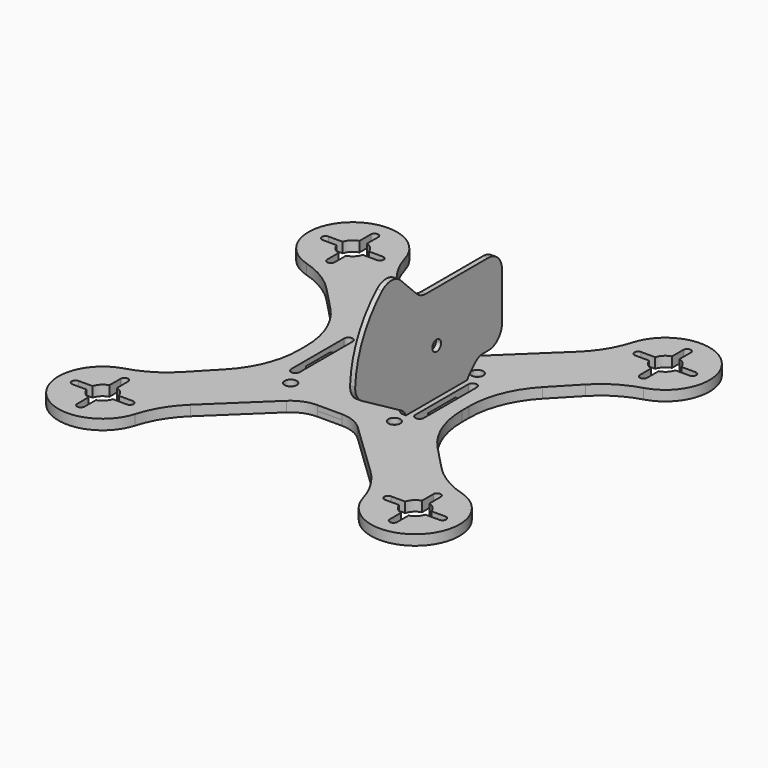
from build123d import *

# Parameters (mm, degrees)
F0_R     = 1.75
F0_W     = 2.5
F0_H     = 22
F0_R_2   = 5
F1_DEPTH = 3
F2_R     = 1.75
F2_R_2   = 8
F2_R_3   = 3.5
F3_DEPTH = 1.5
F4_R     = 1.24999
F6_W     = 11.5
F6_H     = 1.5
F6_R     = 1.6
F7_DEPTH = 1.5


# Not quite as in the source:
# - a fillet or chamfer is up to 0.001 mm smaller than in the source, because OpenCascade refuses the exact size


with BuildPart() as f1:
    # F0 (on Top) → F1 (new body)
    with BuildSketch(Plane.XY):
        with BuildLine():
            ThreePointArc((38.0929628562, 26.4985966632), (43.3866280041, 30.7474383597), (49.5996537841, 33.4812739649))
            ThreePointArc((49.5996537841, 33.4812739649), (55.1543289326, 55.1543289326), (33.4812739649, 49.5996537841))
            ThreePointArc((33.4812739649, 49.5996537841), (30.7474383597, 43.3866280041), (26.4985966632, 38.0929628562))
            Line((26.4985966632, 38.0929628562), (10.4972371837, 22.7761088685))
            ThreePointArc((10.4972371837, 22.7761088685), (7.3080296231, 20.7199431221), (3.5823693672, 20))
            Line((3.5823693672, 20), (-3.5823693672, 20))
            ThreePointArc((-3.5823693672, 20), (-7.3080296231, 20.7199431221), (-10.4972371837, 22.7761088685))
            Line((-10.4972371837, 22.7761088685), (-26.4985966632, 38.0929628562))
            ThreePointArc((-26.4985966632, 38.0929628562), (-30.7474383597, 43.3866280041), (-33.4812739649, 49.5996537841))
            ThreePointArc((-33.4812739649, 49.5996537841), (-55.1543289326, 55.1543289326), (-49.5996537841, 33.4812739649))
            ThreePointArc((-49.5996537841, 33.4812739649), (-43.3866280041, 30.7474383597), (-38.0929628562, 26.4985966632))
            Line((-38.0929628562, 26.4985966632), (-31.217883058, 19.3162716643))
            ThreePointArc((-31.217883058, 19.3162716643), (-25.8718521174, 11.0243320067), (-24, 1.3376153414))
            Line((-24, 1.3376153414), (-24, -1.3376153414))
            ThreePointArc((-24, -1.3376153414), (-25.8718521174, -11.0243320067), (-31.217883058, -19.3162716643))
            Line((-31.217883058, -19.3162716643), (-38.0929628562, -26.4985966632))
            ThreePointArc((-38.0929628562, -26.4985966632), (-43.3866280041, -30.7474383597), (-49.5996537841, -33.4812739649))
            ThreePointArc((-49.5996537841, -33.4812739649), (-55.1543289326, -55.1543289326), (-33.4812739649, -49.5996537841))
            ThreePointArc((-33.4812739649, -49.5996537841), (-30.7474383597, -43.3866280041), (-26.4985966632, -38.0929628562))
            Line((-26.4985966632, -38.0929628562), (-10.4972371837, -22.7761088685))
            ThreePointArc((-10.4972371837, -22.7761088685), (-7.3080296231, -20.7199431221), (-3.5823693672, -20))
            Line((-3.5823693672, -20), (3.5823693672, -20))
            ThreePointArc((3.5823693672, -20), (7.3080296231, -20.7199431221), (10.4972371837, -22.7761088685))
            Line((10.4972371837, -22.7761088685), (26.4985966632, -38.0929628562))
            ThreePointArc((26.4985966632, -38.0929628562), (30.7474383597, -43.3866280041), (33.4812739649, -49.5996537841))
            ThreePointArc((33.4812739649, -49.5996537841), (55.1543289326, -55.1543289326), (49.5996537841, -33.4812739649))
            ThreePointArc((49.5996537841, -33.4812739649), (43.3866280041, -30.7474383597), (38.0929628562, -26.4985966632))
            Line((38.0929628562, -26.4985966632), (31.217883058, -19.3162716643))
            ThreePointArc((31.217883058, -19.3162716643), (25.8718521174, -11.0243320067), (24, -1.3376153414))
            Line((24, -1.3376153414), (24, 1.3376153414))
            ThreePointArc((24, 1.3376153414), (25.8718521174, 11.0243320067), (31.217883058, 19.3162716643))
            Line((31.217883058, 19.3162716643), (38.0929628562, 26.4985966632))
        make_face()
        with BuildLine():
            Line((-42.1161638725, -44.8619407771), (-37.9619407771, -44.8619407771))
            ThreePointArc((-37.9619407771, -44.8619407771), (-36.8619407771, -45.9619407771), (-37.9619407771, -47.0619407771))
            Line((-37.9619407771, -47.0619407771), (-42.1161638725, -47.0619407771))
            ThreePointArc((-42.1161638725, -47.0619407771), (-43.1335136524, -48.7903679019), (-44.8619407771, -49.8077176817))
            Line((-44.8619407771, -49.8077176817), (-44.8619407771, -53.9619407771))
            ThreePointArc((-44.8619407771, -53.9619407771), (-45.9619407771, -55.0619407771), (-47.0619407771, -53.9619407771))
            Line((-47.0619407771, -53.9619407771), (-47.0619407771, -49.8077176817))
            ThreePointArc((-47.0619407771, -49.8077176817), (-48.7903679019, -48.7903679019), (-49.8077176817, -47.0619407771))
            Line((-49.8077176817, -47.0619407771), (-53.9619407771, -47.0619407771))
            ThreePointArc((-53.9619407771, -47.0619407771), (-55.0619407771, -45.9619407771), (-53.9619407771, -44.8619407771))
            Line((-53.9619407771, -44.8619407771), (-49.8077176817, -44.8619407771))
            ThreePointArc((-49.8077176817, -44.8619407771), (-48.7903679019, -43.1335136524), (-47.0619407771, -42.1161638725))
            Line((-47.0619407771, -42.1161638725), (-47.0619407771, -37.9619407771))
            ThreePointArc((-47.0619407771, -37.9619407771), (-45.9619407771, -36.8619407771), (-44.8619407771, -37.9619407771))
            Line((-44.8619407771, -37.9619407771), (-44.8619407771, -42.1161638725))
            ThreePointArc((-44.8619407771, -42.1161638725), (-43.1335136524, -43.1335136524), (-42.1161638725, -44.8619407771))
        make_face(mode=Mode.SUBTRACT)
        with Locations((-15.25, -15.25)):
            Circle(F0_R, mode=Mode.SUBTRACT)
        with BuildLine():
            Line((44.8619407771, -42.1161638725), (44.8619407771, -37.9619407771))
            ThreePointArc((44.8619407771, -37.9619407771), (45.9619407771, -36.8619407771), (47.0619407771, -37.9619407771))
            Line((47.0619407771, -37.9619407771), (47.0619407771, -42.1161638725))
            ThreePointArc((47.0619407771, -42.1161638725), (48.7903679019, -43.1335136524), (49.8077176817, -44.8619407771))
            Line((49.8077176817, -44.8619407771), (53.9619407771, -44.8619407771))
            ThreePointArc((53.9619407771, -44.8619407771), (55.0619407771, -45.9619407771), (53.9619407771, -47.0619407771))
            Line((53.9619407771, -47.0619407771), (49.8077176817, -47.0619407771))
            ThreePointArc((49.8077176817, -47.0619407771), (48.7903679019, -48.7903679019), (47.0619407771, -49.8077176817))
            Line((47.0619407771, -49.8077176817), (47.0619407771, -53.9619407771))
            ThreePointArc((47.0619407771, -53.9619407771), (45.9619407771, -55.0619407771), (44.8619407771, -53.9619407771))
            Line((44.8619407771, -53.9619407771), (44.8619407771, -49.8077176817))
            ThreePointArc((44.8619407771, -49.8077176817), (43.1335136524, -48.7903679019), (42.1161638725, -47.0619407771))
            Line((42.1161638725, -47.0619407771), (37.9619407771, -47.0619407771))
            ThreePointArc((37.9619407771, -47.0619407771), (36.8619407771, -45.9619407771), (37.9619407771, -44.8619407771))
            Line((37.9619407771, -44.8619407771), (42.1161638725, -44.8619407771))
            ThreePointArc((42.1161638725, -44.8619407771), (43.1335136524, -43.1335136524), (44.8619407771, -42.1161638725))
        make_face(mode=Mode.SUBTRACT)
        with Locations((15.25, -15.25)):
            Circle(F0_R, mode=Mode.SUBTRACT)
        with Locations((-18.25, 0)):
            Rectangle(F0_W, F0_H, mode=Mode.SUBTRACT)
        with Locations((-15.25, 15.25)):
            Circle(F0_R, mode=Mode.SUBTRACT)
        with BuildLine():
            Line((-44.8619407771, 42.1161638725), (-44.8619407771, 37.9619407771))
            ThreePointArc((-44.8619407771, 37.9619407771), (-45.9619407771, 36.8619407771), (-47.0619407771, 37.9619407771))
            Line((-47.0619407771, 37.9619407771), (-47.0619407771, 42.1161638725))
            ThreePointArc((-47.0619407771, 42.1161638725), (-48.7903679019, 43.1335136524), (-49.8077176817, 44.8619407771))
            Line((-49.8077176817, 44.8619407771), (-53.9619407771, 44.8619407771))
            ThreePointArc((-53.9619407771, 44.8619407771), (-55.0619407771, 45.9619407771), (-53.9619407771, 47.0619407771))
            Line((-53.9619407771, 47.0619407771), (-49.8077176817, 47.0619407771))
            ThreePointArc((-49.8077176817, 47.0619407771), (-48.7903679019, 48.7903679019), (-47.0619407771, 49.8077176817))
            Line((-47.0619407771, 49.8077176817), (-47.0619407771, 53.9619407771))
            ThreePointArc((-47.0619407771, 53.9619407771), (-45.9619407771, 55.0619407771), (-44.8619407771, 53.9619407771))
            Line((-44.8619407771, 53.9619407771), (-44.8619407771, 49.8077176817))
            ThreePointArc((-44.8619407771, 49.8077176817), (-43.1335136524, 48.7903679019), (-42.1161638725, 47.0619407771))
            Line((-42.1161638725, 47.0619407771), (-37.9619407771, 47.0619407771))
            ThreePointArc((-37.9619407771, 47.0619407771), (-36.8619407771, 45.9619407771), (-37.9619407771, 44.8619407771))
            Line((-37.9619407771, 44.8619407771), (-42.1161638725, 44.8619407771))
            ThreePointArc((-42.1161638725, 44.8619407771), (-43.1335136524, 43.1335136524), (-44.8619407771, 42.1161638725))
        make_face(mode=Mode.SUBTRACT)
        Circle(F0_R_2, mode=Mode.SUBTRACT)
        with Locations((18.25, 0)):
            Rectangle(F0_W, F0_H, mode=Mode.SUBTRACT)
        with Locations((15.25, 15.25)):
            Circle(F0_R, mode=Mode.SUBTRACT)
        with BuildLine():
            ThreePointArc((42.1161638725, 47.0619407771), (43.1335136524, 48.7903679019), (44.8619407771, 49.8077176817))
            Line((44.8619407771, 49.8077176817), (44.8619407771, 53.9619407771))
            ThreePointArc((44.8619407771, 53.9619407771), (45.9619407771, 55.0619407771), (47.0619407771, 53.9619407771))
            Line((47.0619407771, 53.9619407771), (47.0619407771, 49.8077176817))
            ThreePointArc((47.0619407771, 49.8077176817), (48.7903679019, 48.7903679019), (49.8077176817, 47.0619407771))
            Line((49.8077176817, 47.0619407771), (53.9619407771, 47.0619407771))
            ThreePointArc((53.9619407771, 47.0619407771), (55.0619407771, 45.9619407771), (53.9619407771, 44.8619407771))
            Line((53.9619407771, 44.8619407771), (49.8077176817, 44.8619407771))
            ThreePointArc((49.8077176817, 44.8619407771), (48.7903679019, 43.1335136524), (47.0619407771, 42.1161638725))
            Line((47.0619407771, 42.1161638725), (47.0619407771, 37.9619407771))
            ThreePointArc((47.0619407771, 37.9619407771), (45.9619407771, 36.8619407771), (44.8619407771, 37.9619407771))
            Line((44.8619407771, 37.9619407771), (44.8619407771, 42.1161638725))
            ThreePointArc((44.8619407771, 42.1161638725), (43.1335136524, 43.1335136524), (42.1161638725, 44.8619407771))
            Line((42.1161638725, 44.8619407771), (37.9619407771, 44.8619407771))
            ThreePointArc((37.9619407771, 44.8619407771), (36.8619407771, 45.9619407771), (37.9619407771, 47.0619407771))
            Line((37.9619407771, 47.0619407771), (42.1161638725, 47.0619407771))
        make_face(mode=Mode.SUBTRACT)
    extrude(amount=F1_DEPTH)

    # F4 (radius 1.25 in the source; OpenCascade refuses exactly that, so slightly less here)
    f4_edges = [f1.edges().sort_by_distance(p)[0] for p in [
        (-19.5, 11, 1.5),
        (-17, 11, 1.5),
        (-19.5, -11, 1.5),
        (-17, -11, 1.5),
        (17, -11, 1.5),
        (19.5, -11, 1.5),
        (17, 11, 1.5),
        (19.5, 11, 1.5),
    ]]
    fillet(f4_edges, radius=F4_R)


with BuildPart() as f3:
    # F2 (on Top) → F3 (new body)
    with BuildSketch(Plane.XY):
        with BuildLine():
            Line((-10.9087121146, 20), (-15, 20))
            ThreePointArc((-15, 20), (-18.5355339059, 18.5355339059), (-20, 15))
            Line((-20, 15), (-20, 13))
            ThreePointArc((-20, 13), (-19.4142135624, 11.5857864376), (-18, 11))
            Line((-18, 11), (-14, 11))
            ThreePointArc((-14, 11), (-13.5, 10.5), (-14, 10))
            Line((-14, 10), (-14, 6))
            ThreePointArc((-14, 6), (-13.5, 5.5), (-14, 5))
            Line((-14, 5), (-18, 5))
            ThreePointArc((-18, 5), (-19.4142135624, 4.4142135624), (-20, 3))
            Line((-20, 3), (-20, -3))
            ThreePointArc((-20, -3), (-19.4142135624, -4.4142135624), (-18, -5))
            Line((-18, -5), (-14, -5))
            ThreePointArc((-14, -5), (-13.5, -5.5), (-14, -6))
            Line((-14, -6), (-14, -10))
            ThreePointArc((-14, -10), (-13.5, -10.5), (-14, -11))
            Line((-14, -11), (-18, -11))
            ThreePointArc((-18, -11), (-19.4142135624, -11.5857864376), (-20, -13))
            Line((-20, -13), (-20, -15))
            ThreePointArc((-20, -15), (-18.5355339059, -18.5355339059), (-15, -20))
            Line((-15, -20), (15, -20))
            ThreePointArc((15, -20), (18.5355339059, -18.5355339059), (20, -15))
            Line((20, -15), (20, -13))
            ThreePointArc((20, -13), (19.4142135624, -11.5857864376), (18, -11))
            Line((18, -11), (14, -11))
            ThreePointArc((14, -11), (13.5, -10.5), (14, -10))
            Line((14, -10), (14, -6))
            ThreePointArc((14, -6), (13.5, -5.5), (14, -5))
            Line((14, -5), (18, -5))
            ThreePointArc((18, -5), (19.4142135624, -4.4142135624), (20, -3))
            Line((20, -3), (20, 3))
            ThreePointArc((20, 3), (19.4142135624, 4.4142135624), (18, 5))
            Line((18, 5), (14, 5))
            ThreePointArc((14, 5), (13.5, 5.5), (14, 6))
            Line((14, 6), (14, 10))
            ThreePointArc((14, 10), (13.5, 10.5), (14, 11))
            Line((14, 11), (18, 11))
            ThreePointArc((18, 11), (19.4142135624, 11.5857864376), (20, 13))
            Line((20, 13), (20, 15))
            ThreePointArc((20, 15), (18.5355339059, 18.5355339059), (15, 20))
            Line((15, 20), (10.9087121146, 20))
            ThreePointArc((10.9087121146, 20), (8.2084034903, 20.7918729423), (6.3634154002, 22.9166666667))
            ThreePointArc((6.3634154002, 22.9166666667), (0, 27), (-6.3634154002, 22.9166666667))
            ThreePointArc((-6.3634154002, 22.9166666667), (-8.2084034903, 20.7918729423), (-10.9087121146, 20))
        make_face()
        with Locations((-15.25, -15.25)):
            Circle(F2_R, mode=Mode.SUBTRACT)
        with Locations((15.25, -15.25)):
            Circle(F2_R, mode=Mode.SUBTRACT)
        Circle(F2_R_2, mode=Mode.SUBTRACT)
        with Locations((-15.25, 15.25)):
            Circle(F2_R, mode=Mode.SUBTRACT)
        with Locations((0, 20)):
            Circle(F2_R_3, mode=Mode.SUBTRACT)
        with Locations((15.25, 15.25)):
            Circle(F2_R, mode=Mode.SUBTRACT)
    extrude(amount=F3_DEPTH)


with BuildPart() as f7:
    # F6 (on offset) → F7 (new body)
    with BuildSketch(Plane.YZ.offset(14)):
        with BuildLine():
            ThreePointArc((-11, 0), (-9.8284271247, -2.8284271247), (-7, -4))
            Line((-7, -4), (7, -4))
            ThreePointArc((7, -4), (9.8284271247, -2.8284271247), (11, 0))
            Line((11, 0), (11, 1.5))
            ThreePointArc((11, 1.5), (11.30448187, 3.0307337295), (12.1715728753, 4.3284271247))
            Line((12.1715728753, 4.3284271247), (14.1715728753, 6.3284271247))
            ThreePointArc((14.1715728753, 6.3284271247), (15.4692662705, 7.19551813), (17, 7.5))
            Line((17, 7.5), (19, 7.5))
            ThreePointArc((19, 7.5), (22.5355339059, 8.9644660941), (24, 12.5))
            Line((24, 12.5), (24, 26.5))
            ThreePointArc((24, 26.5), (22.5355339059, 30.0355339059), (19, 31.5))
            Line((19, 31.5), (-3.9289321881, 31.5))
            ThreePointArc((-3.9289321881, 31.5), (-5.84234935, 31.8806023374), (-7.4644660941, 32.9644660941))
            Line((-7.4644660941, 32.9644660941), (-13.1513400385, 38.6513400385))
            ThreePointArc((-13.1513400385, 38.6513400385), (-16.5504270251, 40.1139440096), (-20.0242487333, 38.838967359))
            ThreePointArc((-20.0242487333, 38.838967359), (-27.1039610544, 29.3598326256), (-29.9682147358, 17.8806178139))
            ThreePointArc((-29.9682147358, 17.8806178139), (-29.3600331805, 15.2508410362), (-27.4735122798, 13.320387826))
            Line((-27.4735122798, 13.320387826), (-13, 4.9641016151))
            ThreePointArc((-13, 4.9641016151), (-11.5358983849, 3.5), (-11, 1.5))
            Line((-11, 1.5), (-11, 0))
        make_face()
        with Locations((0, 0.75)):
            Rectangle(F6_W, F6_H, mode=Mode.SUBTRACT)
        with Locations((0, 16.5)):
            Circle(F6_R, mode=Mode.SUBTRACT)
    extrude(amount=F7_DEPTH)


solid = Compound([f1.part, f3.part, f7.part])
